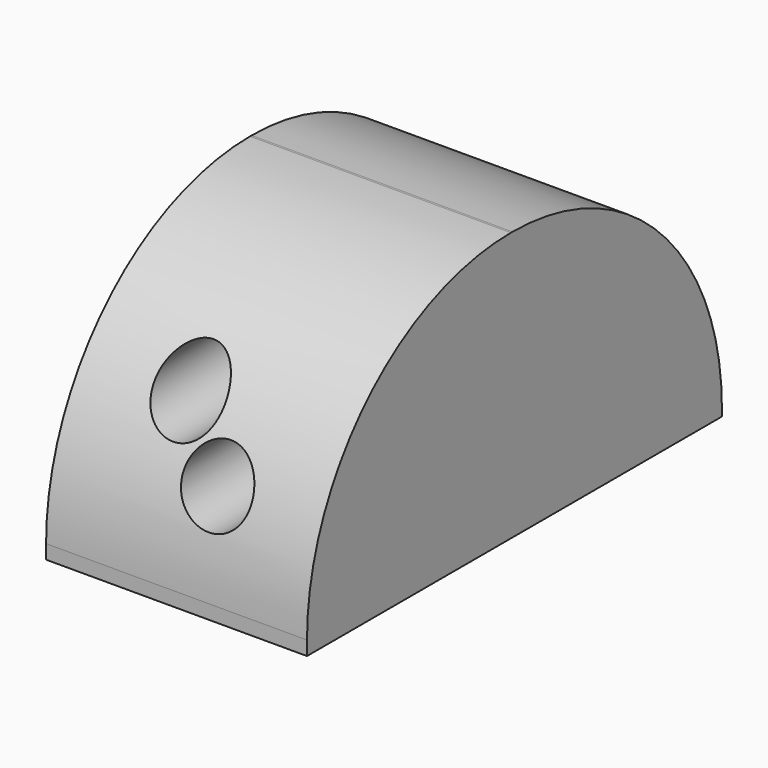
from build123d import *

# Parameters (mm, degrees)
F0_W        = 92.8924418986
F0_H        = 95.79378739
F1_DEPTH    = 98.552
F2_DEPTH    = 86.106
F3_R        = 12.3937050542
F4_DEPTH    = 203.2
F5_R        = 12.4518339151
F6_DEPTH    = 203.2
F7_T1_DEPTH = 546.6680230822
F8_T1_DEPTH = 558.9322279791


# Not quite as in the source:
# - a fillet or chamfer that OpenCascade refuses, or shapes differently, is made with other operations: its cross-section is extruded or revolved along the edge and cut away or added


with BuildPart() as f1:
    # F0 (on Front) → F1 (new body)
    with BuildSketch(Plane.XZ):
        with Locations((-6.0582030565, -12.6477908343)):
            Rectangle(F0_W, F0_H)
    extrude(amount=F1_DEPTH)

    # F2 (add): a face of the model
    f2_faces = [f1.faces().sort_by_distance(p)[0] for p in [
        (-6.0582030565, 0, -12.6477908343),
    ]]
    extrude(f2_faces, amount=F2_DEPTH)

    # F3 (on face) → F4 (cut)
    with BuildSketch(Plane.XZ.offset(98.552)):
        with Locations((-14.8652456701, -2.7690164279)):
            Circle(F3_R)
    extrude(amount=-F4_DEPTH, mode=Mode.SUBTRACT)

    # F5 (on face) → F6 (cut)
    with BuildSketch(Plane.XZ.offset(98.552)):
        with Locations((3.47437663, -22.2978685051)):
            Circle(F5_R)
    extrude(amount=-F6_DEPTH, mode=Mode.SUBTRACT)

    # F7: fillet of radius 90.7551162367 on 1 edges, made by hand

    # F7_s2 → F7_t1 (cut)
    with BuildSketch(Plane.YZ.offset(-279.3922145976)):
        with BuildLine():
            ThreePointArc((-7.7968837633, 35.2491028607), (-71.9704418816, 8.6675447423), (-98.552, -55.506013376))
            Line((-98.552, -55.506013376), (-98.552, 35.2491028607))
            Line((-98.552, 35.2491028607), (-7.7968837633, 35.2491028607))
        make_face()
    extrude(amount=F7_T1_DEPTH, mode=Mode.SUBTRACT)

    # F8: fillet of radius 93.2079572161 on 1 edges, made by hand

    # F8_s2 → F8_t1 (cut)
    with BuildSketch(Plane.YZ.offset(-285.524317046)):
        with BuildLine():
            ThreePointArc((-7.1019572161, 35.2491028607), (58.8060213919, 7.9491242526), (86.106, -57.9588543554))
            Line((86.106, -57.9588543554), (86.106, 35.2491028607))
            Line((86.106, 35.2491028607), (-7.1019572161, 35.2491028607))
        make_face()
    extrude(amount=F8_T1_DEPTH, mode=Mode.SUBTRACT)


solid = f1.part
